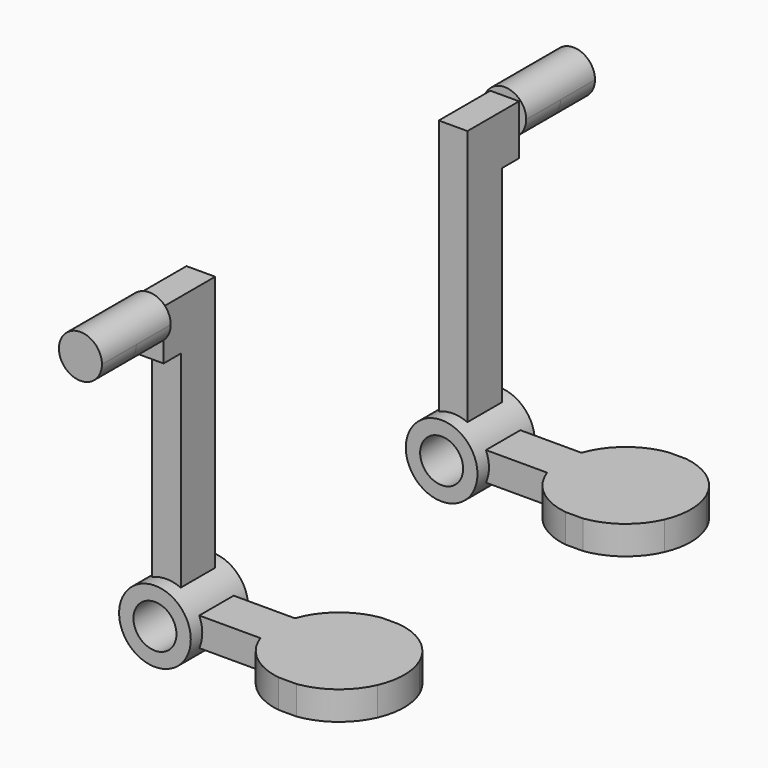
from build123d import *
from build123d import SkipClean  # not in build123d's __all__

# Parameters (mm, degrees)
F0_R           = 6.35
F0_R_2         = 3.81
F1_DEPTH       = 12.7
F4_DEPTH       = 38.1
F5_DEPTH       = 25.4
F5_DEPTH_BACK  = 25.4
F6_W           = 13.8230553448
F6_H           = 5.08
F7_DEPTH       = 7.62
F7_DEPTH_BACK  = 15.24
F8_DEPTH       = 7.62
F9_DEPTH       = 7.62
F11_DEPTH      = 25.4
F12_DEPTH      = 5.08
F14_DEPTH      = 51.2318
F15_DEPTH      = 25.4
F16_W          = 2.54
F16_H          = 8.89
F17_DEPTH      = 11.43
F19_DEPTH      = 7.62
F19_DEPTH_BACK = 7.62
F20_DEPTH      = 7.62


with BuildPart() as f1:
    # F0 (on Front) → F1 (new body)
    with BuildSketch(Plane.XZ):
        Circle(F0_R)
        Circle(F0_R_2, mode=Mode.SUBTRACT)
    extrude(amount=F1_DEPTH)

    # F3 (on Right) → F4 (join)
    with BuildSketch(Plane.YZ):
        Polygon((-2.54, -2.54), (-2.54, 0), (-2.54, 2.54), (-10.16, 2.54), (-10.16, 0), (-10.16, -2.54), align=None)
    extrude(amount=F4_DEPTH)

    # F0 (on Front) → F5 (cut, two sides)
    with BuildSketch(Plane.XZ) as f5_sk:
        Circle(F0_R_2)
    extrude(amount=F5_DEPTH, mode=Mode.SUBTRACT)
    extrude(f5_sk.sketch, amount=-F5_DEPTH_BACK, mode=Mode.SUBTRACT)

    # F6 (on face) → F7 (join, two sides)
    with BuildSketch(Plane.XZ.offset(10.16)) as f7_sk:
        with Locations((31.1884723276, 0)):
            Rectangle(F6_W, F6_H)
    extrude(amount=F7_DEPTH)
    extrude(f7_sk.sketch, amount=-F7_DEPTH_BACK)

    # F8 (add): a face of the model
    f8_faces = [f1.faces().sort_by_distance(p)[0] for p in [
        (24.2769446552, -13.97, 0),
    ]]
    extrude(f8_faces, amount=F8_DEPTH)

    # F9 (add): a face of the model
    f9_faces = [f1.faces().sort_by_distance(p)[0] for p in [
        (24.2769446552, 1.27, 0),
    ]]
    extrude(f9_faces, amount=F9_DEPTH)

    # F10 (on face) → F11 (cut)
    with BuildSketch(Plane.XY.offset(2.54)):
        with BuildLine():
            ThreePointArc((25.9835010893, -17.78), (20.2469210754, -15.2836758241), (16.6569446552, -10.16))
            Line((16.6569446552, -10.16), (16.6569446552, -17.78))
            Line((16.6569446552, -17.78), (25.9835010893, -17.78))
        make_face()
        with BuildLine():
            Line((16.6569446552, 5.08), (16.6569446552, -2.54))
            ThreePointArc((16.6569446552, -2.54), (20.2469210754, 2.5836758241), (25.9835010893, 5.08))
            Line((25.9835010893, 5.08), (16.6569446552, 5.08))
        make_face()
        with BuildLine():
            Line((38.1, 5.08), (29.1083570088, 5.08))
            ThreePointArc((29.1083570088, 5.08), (34.4861831348, 2.8651480918), (38.1, -1.6919244863))
            Line((38.1, -1.6919244863), (38.1, 5.08))
        make_face()
        with BuildLine():
            Line((38.1, -17.78), (38.1, -11.0080755137))
            ThreePointArc((38.1, -11.0080755137), (34.4861831348, -15.5651480918), (29.1083570088, -17.78))
            Line((29.1083570088, -17.78), (38.1, -17.78))
        make_face()
    extrude(amount=-F11_DEPTH, mode=Mode.SUBTRACT)

    # F10 (on face) → F12 (join)
    with BuildSketch(Plane.XY.offset(2.54)):
        with BuildLine():
            ThreePointArc((38.1, -11.0080755137), (39.0822231303, -6.35), (38.1, -1.6919244863))
            Line((38.1, -1.6919244863), (38.1, -11.0080755137))
        make_face()
    with SkipClean():  # cleaning this boolean's faces spoils the solid; the shape is the same uncleaned
        extrude(amount=-F12_DEPTH)

    # F13 (on Top) → F14 (join)
    with BuildSketch(Plane.XY):
        Polygon((2.54, -2.54), (0, -2.54), (-2.54, -2.54), (-2.54, -10.16), (0, -10.16), (2.54, -10.16), align=None)
    extrude(amount=F14_DEPTH)

    # F0 (on Front) → F15 (cut)
    with BuildSketch(Plane.XZ):
        Circle(F0_R_2)
    extrude(amount=F15_DEPTH, mode=Mode.SUBTRACT)

    # F16 (on face) → F17 (join)
    with BuildSketch(Plane.XZ.offset(10.16)):
        with Locations((-1.27, 46.7868)):
            Rectangle(F16_W, F16_H)
        with Locations((1.27, 46.7868)):
            Rectangle(F16_W, F16_H)
    extrude(amount=F17_DEPTH)

    # F18 (on face) → F19 (join, two sides)
    with BuildSketch(Plane.XZ.offset(21.59)) as f19_sk:
        with BuildLine():
            Line((-2.54, 51.2318), (-2.54, 45.9789936686))
            ThreePointArc((-2.54, 45.9789936686), (-1.359492162, 45.2596033124), (0, 45.0088))
            ThreePointArc((0, 45.0088), (1.359492162, 45.2596033124), (2.54, 45.9789936686))
            Line((2.54, 45.9789936686), (2.54, 51.2318))
            Line((2.54, 51.2318), (-2.54, 51.2318))
        make_face()
        with BuildLine():
            ThreePointArc((2.54, 45.9789936686), (3.4780382402, 47.2633740133), (3.81, 48.8188))
            ThreePointArc((3.81, 48.8188), (-1.5554259867, 52.2968382402), (-2.54, 45.9789936686))
            Line((-2.54, 45.9789936686), (-2.54, 51.2318))
            Line((-2.54, 51.2318), (2.54, 51.2318))
            Line((2.54, 51.2318), (2.54, 45.9789936686))
        make_face()
    extrude(amount=F19_DEPTH)
    extrude(f19_sk.sketch, amount=-F19_DEPTH_BACK)

    # F20 (cut): a face of the model
    f20_faces = [f1.faces().sort_by_distance(p)[0] for p in [
        (0, -21.59, 43.8411826896),
    ]]
    extrude(f20_faces, amount=-F20_DEPTH, mode=Mode.SUBTRACT)


with BuildPart() as f22_1:
    # F22: instance of F1
    add(f1.part.mirror(Plane.XZ.offset(-25.4)), clean=False)


solid = Compound([f1.part, f22_1.part])
